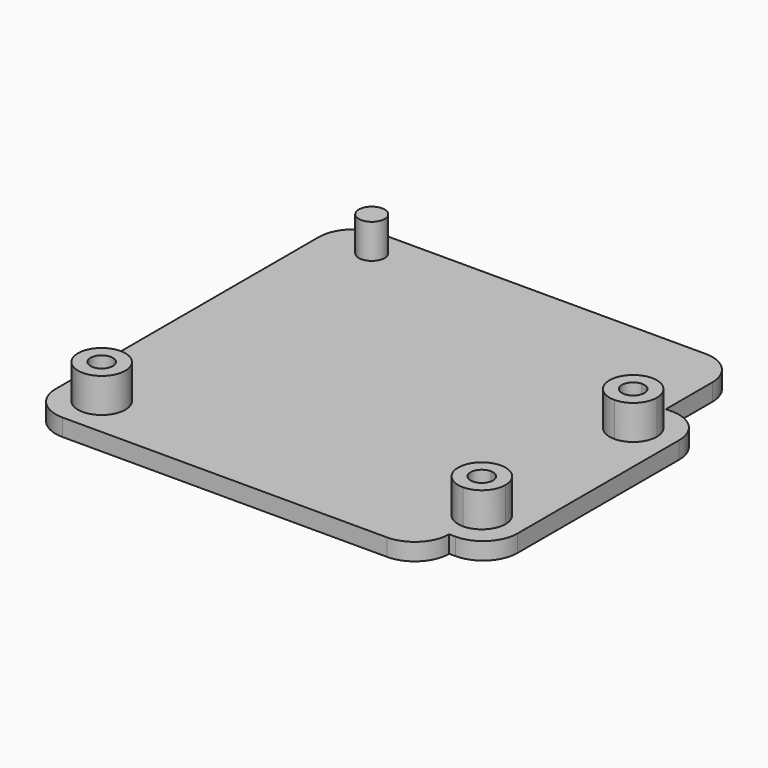
from build123d import *

# Parameters (mm, degrees)
F1_R     = 3.4925
F1_R_2   = 1.905
F2_DEPTH = 2.54
F1_R_3   = 1.651
F3_DEPTH = 7.62
F4_R     = 5.07999


# Not quite as in the source:
# - a fillet or chamfer is up to 0.001 mm smaller than in the source, because OpenCascade refuses the exact size


with BuildPart() as f2:
    # F1 (on Top) → F2 (new body)
    with BuildSketch(Plane.XY):
        with BuildLine():
            ThreePointArc((25.4, -22.5425), (21.9075, -19.05), (25.4, -15.5575))
            Line((25.4, -15.5575), (25.4, 5.3975))
            ThreePointArc((25.4, 5.3975), (21.9075, 8.89), (25.4, 12.3825))
            Line((25.4, 12.3825), (25.4, 14.9225))
            Line((25.4, 14.9225), (25.4, 28.575))
            Line((25.4, 28.575), (-32.7025, 28.575))
            Line((-32.7025, 28.575), (-32.7025, -30.1625))
            Line((-32.7025, -30.1625), (25.4, -30.1625))
            Line((25.4, -30.1625), (25.4, -25.0825))
            Line((25.4, -25.0825), (25.4, -22.5425))
        make_face()
        with Locations((-26.67, -24.13)):
            Circle(F1_R, mode=Mode.SUBTRACT)
        with Locations((-25.4, 24.13)):
            Circle(F1_R_2, mode=Mode.SUBTRACT)
        with BuildLine():
            ThreePointArc((25.4, -15.5575), (27.8695704333, -16.5804295667), (28.8925, -19.05))
            ThreePointArc((28.8925, -19.05), (27.8695704333, -21.5195704333), (25.4, -22.5425))
            Line((25.4, -22.5425), (25.4, -25.0825))
            Line((25.4, -25.0825), (31.4325, -25.0825))
            Line((31.4325, -25.0825), (31.4325, 14.9225))
            Line((31.4325, 14.9225), (25.4, 14.9225))
            Line((25.4, 14.9225), (25.4, 12.3825))
            ThreePointArc((25.4, 12.3825), (27.8695704333, 11.3595704333), (28.8925, 8.89))
            ThreePointArc((28.8925, 8.89), (27.8695704333, 6.4204295667), (25.4, 5.3975))
            Line((25.4, 5.3975), (25.4, -15.5575))
        make_face()
    extrude(amount=F2_DEPTH)

    # F1 (on Top) → F3 (join)
    with BuildSketch(Plane.XY):
        with Locations((-26.67, -24.13)):
            Circle(F1_R)
        with Locations((-26.67, -24.13)):
            Circle(F1_R_3, mode=Mode.SUBTRACT)
        with Locations((-25.4, 24.13)):
            Circle(F1_R_2)
        with BuildLine():
            ThreePointArc((25.4, 12.3825), (21.9075, 8.89), (25.4, 5.3975))
            Line((25.4, 5.3975), (25.4, 7.239))
            ThreePointArc((25.4, 7.239), (23.749, 8.89), (25.4, 10.541))
            Line((25.4, 10.541), (25.4, 12.3825))
        make_face()
        with BuildLine():
            Line((25.4, 7.239), (25.4, 5.3975))
            ThreePointArc((25.4, 5.3975), (27.8695704333, 6.4204295667), (28.8925, 8.89))
            ThreePointArc((28.8925, 8.89), (27.8695704333, 11.3595704333), (25.4, 12.3825))
            Line((25.4, 12.3825), (25.4, 10.541))
            ThreePointArc((25.4, 10.541), (26.5674332957, 10.0574332957), (27.051, 8.89))
            ThreePointArc((27.051, 8.89), (26.5674332957, 7.7225667043), (25.4, 7.239))
        make_face()
        with BuildLine():
            Line((25.4, -17.399), (25.4, -15.5575))
            ThreePointArc((25.4, -15.5575), (21.9075, -19.05), (25.4, -22.5425))
            Line((25.4, -22.5425), (25.4, -20.701))
            ThreePointArc((25.4, -20.701), (23.749, -19.05), (25.4, -17.399))
        make_face()
        with BuildLine():
            ThreePointArc((25.4, -22.5425), (27.8695704333, -21.5195704333), (28.8925, -19.05))
            ThreePointArc((28.8925, -19.05), (27.8695704333, -16.5804295667), (25.4, -15.5575))
            Line((25.4, -15.5575), (25.4, -17.399))
            ThreePointArc((25.4, -17.399), (26.5674332957, -17.8825667043), (27.051, -19.05))
            ThreePointArc((27.051, -19.05), (26.5674332957, -20.2174332957), (25.4, -20.701))
            Line((25.4, -20.701), (25.4, -22.5425))
        make_face()
    extrude(amount=F3_DEPTH)

    # F4 (radius 5.08 in the source; OpenCascade refuses exactly that, so slightly less here)
    f4_edges = [f2.edges().sort_by_distance(p)[0] for p in [
        (-32.7025, -30.1625, 1.27),
        (25.4, -30.1625, 1.27),
        (31.4325, -25.0825, 1.27),
        (31.4325, 14.9225, 1.27),
        (25.4, 28.575, 1.27),
        (-32.7025, 28.575, 1.27),
    ]]
    fillet(f4_edges, radius=F4_R)


solid = f2.part
